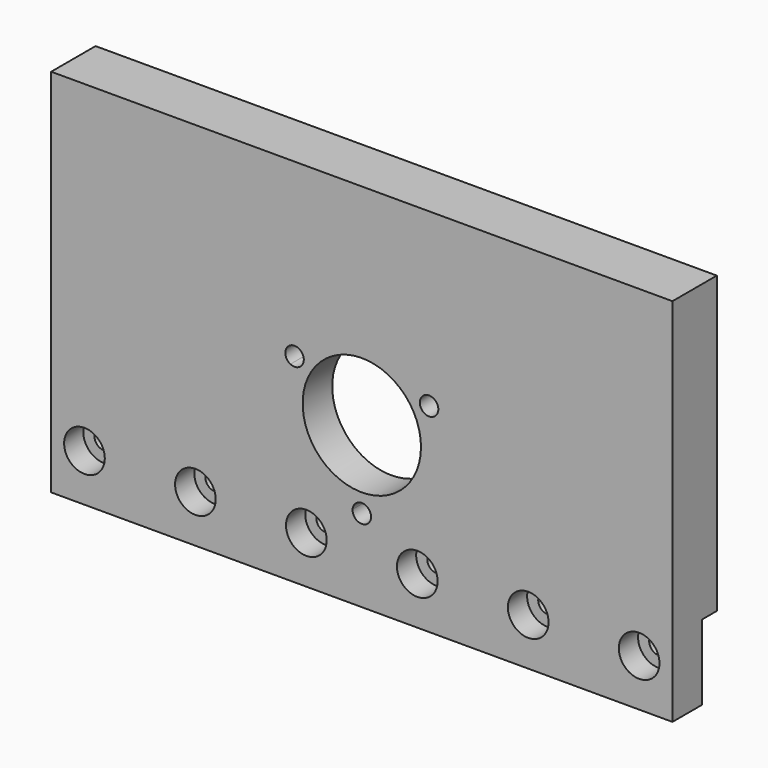
from build123d import *

# Parameters (mm, degrees)
F0_R     = 16
F0_R_2   = 2.5
F1_DEPTH = 15
F2_DEPTH = 5
F3_R     = 5.5
F3_R_2   = 2.5
F4_DEPTH = 6.5


# Not quite as in the source:
# - a feature names something its author has since deleted; it is built from what else it names


with BuildPart() as f1:
    # F0 (on Front) → F1 (new body)
    with BuildSketch(Plane.XZ):
        with BuildLine():
            ThreePointArc((139.0482066844, -68.5256164076), (148.1685102123, -58.5964356365), (151.4733932528, -45.5256164076))
            ThreePointArc((151.4733932528, -45.5256164076), (110.9025740239, -21.3304994481), (108.8985798211, -68.5256164076))
            ThreePointArc((108.8985798211, -68.5256164076), (123.9733932528, -73.0256164076), (139.0482066844, -68.5256164076))
        make_face()
        with BuildLine():
            ThreePointArc((104.6679489936, -37.2612457748), (103.6217962638, -33.7756164076), (107.1635162088, -32.9387965643))
            ThreePointArc((107.1635162088, -32.9387965643), (123.9733932528, -24.5256164076), (140.7832702967, -32.9387965643))
            ThreePointArc((140.7832702967, -32.9387965643), (143.344907515, -32.8242939541), (144.6599267322, -35.0256164076))
            ThreePointArc((144.6599267322, -35.0256164076), (144.2868114199, -36.3395271829), (143.2788375119, -37.2612457748))
            ThreePointArc((143.2788375119, -37.2612457748), (144.5453927842, -41.307460972), (144.9733932528, -45.5256164076))
            ThreePointArc((144.9733932528, -45.5256164076), (139.6801897358, -59.4646459377), (126.468960468, -66.3768068838))
            ThreePointArc((126.468960468, -66.3768068838), (126.4722848108, -66.4511786418), (126.4733932528, -66.5256164076))
            ThreePointArc((126.4733932528, -66.5256164076), (123.8989554869, -69.0245079657), (121.4778260376, -66.3768068838))
            ThreePointArc((121.4778260376, -66.3768068838), (105.7868597733, -56.0256164076), (104.6679489936, -37.2612457748))
        make_face(mode=Mode.SUBTRACT)
        with BuildLine():
            ThreePointArc((107.1635162088, -32.9387965643), (107.9881822268, -33.8406356249), (108.2868597733, -35.0256164076))
            ThreePointArc((108.2868597733, -35.0256164076), (107.1007705486, -37.1525010953), (104.6679489936, -37.2612457748))
            ThreePointArc((104.6679489936, -37.2612457748), (105.7868597733, -56.0256164076), (121.4778260376, -66.3768068838))
            ThreePointArc((121.4778260376, -66.3768068838), (123.9733932528, -64.0256164076), (126.468960468, -66.3768068838))
            ThreePointArc((126.468960468, -66.3768068838), (139.6801897358, -59.4646459377), (144.9733932528, -45.5256164076))
            ThreePointArc((144.9733932528, -45.5256164076), (144.5453927842, -41.307460972), (143.2788375119, -37.2612457748))
            ThreePointArc((143.2788375119, -37.2612457748), (139.9948632228, -36.2756164076), (140.7832702967, -32.9387965643))
            ThreePointArc((140.7832702967, -32.9387965643), (123.9733932528, -24.5256164076), (107.1635162088, -32.9387965643))
        make_face()
        with Locations((123.9733932528, -45.5256164076)):
            Circle(F0_R, mode=Mode.SUBTRACT)
        with BuildLine():
            ThreePointArc((108.8985798211, -68.5256164076), (110.9025740239, -21.3304994481), (151.4733932528, -45.5256164076))
            ThreePointArc((151.4733932528, -45.5256164076), (148.1685102123, -58.5964356365), (139.0482066844, -68.5256164076))
            Line((139.0482066844, -68.5256164076), (207.9733932528, -68.5256164076))
            Line((207.9733932528, -68.5256164076), (207.9733932528, 11.3154806698))
            Line((207.9733932528, 11.3154806698), (39.9733932528, 11.3154806698))
            Line((39.9733932528, 11.3154806698), (39.9733932528, -68.5256164076))
            Line((39.9733932528, -68.5256164076), (108.8985798211, -68.5256164076))
        make_face()
        with BuildLine():
            ThreePointArc((139.0482066844, -68.5256164076), (123.9733932528, -73.0256164076), (108.8985798211, -68.5256164076))
            Line((108.8985798211, -68.5256164076), (39.9733932528, -68.5256164076))
            Line((39.9733932528, -68.5256164076), (39.9733932528, -88.8428396075))
            Line((39.9733932528, -88.8428396075), (207.9733932528, -88.8428396075))
            Line((207.9733932528, -88.8428396075), (207.9733932528, -68.5256164076))
            Line((207.9733932528, -68.5256164076), (139.0482066844, -68.5256164076))
        make_face()
        with Locations((48.9733932528, -76.0256164076)):
            Circle(F0_R_2, mode=Mode.SUBTRACT)
        with Locations((78.9733932528, -76.0256164076)):
            Circle(F0_R_2, mode=Mode.SUBTRACT)
        with Locations((108.9733932528, -76.0256164076)):
            Circle(F0_R_2, mode=Mode.SUBTRACT)
        with Locations((138.9733932528, -76.0256164076)):
            Circle(F0_R_2, mode=Mode.SUBTRACT)
        with Locations((168.9733932528, -76.0256164076)):
            Circle(F0_R_2, mode=Mode.SUBTRACT)
        with Locations((198.9733932528, -76.0256164076)):
            Circle(F0_R_2, mode=Mode.SUBTRACT)
    extrude(amount=F1_DEPTH)

    # F0 (on Front) → F2 (cut)
    with BuildSketch(Plane.XZ):
        with BuildLine():
            ThreePointArc((139.0482066844, -68.5256164076), (148.1685102123, -58.5964356365), (151.4733932528, -45.5256164076))
            ThreePointArc((151.4733932528, -45.5256164076), (110.9025740239, -21.3304994481), (108.8985798211, -68.5256164076))
            ThreePointArc((108.8985798211, -68.5256164076), (123.9733932528, -73.0256164076), (139.0482066844, -68.5256164076))
        make_face()
        with BuildLine():
            ThreePointArc((104.6679489936, -37.2612457748), (103.6217962638, -33.7756164076), (107.1635162088, -32.9387965643))
            ThreePointArc((107.1635162088, -32.9387965643), (123.9733932528, -24.5256164076), (140.7832702967, -32.9387965643))
            ThreePointArc((140.7832702967, -32.9387965643), (143.344907515, -32.8242939541), (144.6599267322, -35.0256164076))
            ThreePointArc((144.6599267322, -35.0256164076), (144.2868114199, -36.3395271829), (143.2788375119, -37.2612457748))
            ThreePointArc((143.2788375119, -37.2612457748), (144.5453927842, -41.307460972), (144.9733932528, -45.5256164076))
            ThreePointArc((144.9733932528, -45.5256164076), (139.6801897358, -59.4646459377), (126.468960468, -66.3768068838))
            ThreePointArc((126.468960468, -66.3768068838), (126.4722848108, -66.4511786418), (126.4733932528, -66.5256164076))
            ThreePointArc((126.4733932528, -66.5256164076), (123.8989554869, -69.0245079657), (121.4778260376, -66.3768068838))
            ThreePointArc((121.4778260376, -66.3768068838), (105.7868597733, -56.0256164076), (104.6679489936, -37.2612457748))
        make_face(mode=Mode.SUBTRACT)
        with BuildLine():
            ThreePointArc((107.1635162088, -32.9387965643), (107.9881822268, -33.8406356249), (108.2868597733, -35.0256164076))
            ThreePointArc((108.2868597733, -35.0256164076), (107.1007705486, -37.1525010953), (104.6679489936, -37.2612457748))
            ThreePointArc((104.6679489936, -37.2612457748), (105.7868597733, -56.0256164076), (121.4778260376, -66.3768068838))
            ThreePointArc((121.4778260376, -66.3768068838), (123.9733932528, -64.0256164076), (126.468960468, -66.3768068838))
            ThreePointArc((126.468960468, -66.3768068838), (139.6801897358, -59.4646459377), (144.9733932528, -45.5256164076))
            ThreePointArc((144.9733932528, -45.5256164076), (144.5453927842, -41.307460972), (143.2788375119, -37.2612457748))
            ThreePointArc((143.2788375119, -37.2612457748), (139.9948632228, -36.2756164076), (140.7832702967, -32.9387965643))
            ThreePointArc((140.7832702967, -32.9387965643), (123.9733932528, -24.5256164076), (107.1635162088, -32.9387965643))
        make_face()
        with Locations((123.9733932528, -45.5256164076)):
            Circle(F0_R, mode=Mode.SUBTRACT)
        with BuildLine():
            ThreePointArc((139.0482066844, -68.5256164076), (123.9733932528, -73.0256164076), (108.8985798211, -68.5256164076))
            Line((108.8985798211, -68.5256164076), (39.9733932528, -68.5256164076))
            Line((39.9733932528, -68.5256164076), (39.9733932528, -88.8428396075))
            Line((39.9733932528, -88.8428396075), (207.9733932528, -88.8428396075))
            Line((207.9733932528, -88.8428396075), (207.9733932528, -68.5256164076))
            Line((207.9733932528, -68.5256164076), (139.0482066844, -68.5256164076))
        make_face()
        with Locations((48.9733932528, -76.0256164076)):
            Circle(F0_R_2, mode=Mode.SUBTRACT)
        with Locations((78.9733932528, -76.0256164076)):
            Circle(F0_R_2, mode=Mode.SUBTRACT)
        with Locations((108.9733932528, -76.0256164076)):
            Circle(F0_R_2, mode=Mode.SUBTRACT)
        with Locations((138.9733932528, -76.0256164076)):
            Circle(F0_R_2, mode=Mode.SUBTRACT)
        with Locations((168.9733932528, -76.0256164076)):
            Circle(F0_R_2, mode=Mode.SUBTRACT)
        with Locations((198.9733932528, -76.0256164076)):
            Circle(F0_R_2, mode=Mode.SUBTRACT)
    extrude(amount=F2_DEPTH, mode=Mode.SUBTRACT)

    # F3 (on face) → F4 (cut)
    with BuildSketch(Plane.XZ.offset(15)):
        with Locations((198.9733932528, -76.0256164076)):
            Circle(F3_R)
        with Locations((198.9733932528, -76.0256164076)):
            Circle(F3_R_2, mode=Mode.SUBTRACT)
        with Locations((168.9733932528, -76.0256164076)):
            Circle(F3_R)
        with Locations((168.9733932528, -76.0256164076)):
            Circle(F3_R_2, mode=Mode.SUBTRACT)
        with Locations((138.9733932528, -76.0256164076)):
            Circle(F3_R)
        with Locations((138.9733932528, -76.0256164076)):
            Circle(F3_R_2, mode=Mode.SUBTRACT)
        with Locations((108.9733932528, -76.0256164076)):
            Circle(F3_R)
        with Locations((108.9733932528, -76.0256164076)):
            Circle(F3_R_2, mode=Mode.SUBTRACT)
        with Locations((78.9733932528, -76.0256164076)):
            Circle(F3_R)
        with Locations((78.9733932528, -76.0256164076)):
            Circle(F3_R_2, mode=Mode.SUBTRACT)
        with Locations((48.9733932528, -76.0256164076)):
            Circle(F3_R)
        with Locations((48.9733932528, -76.0256164076)):
            Circle(F3_R_2, mode=Mode.SUBTRACT)
    extrude(amount=-F4_DEPTH, mode=Mode.SUBTRACT)


solid = f1.part
